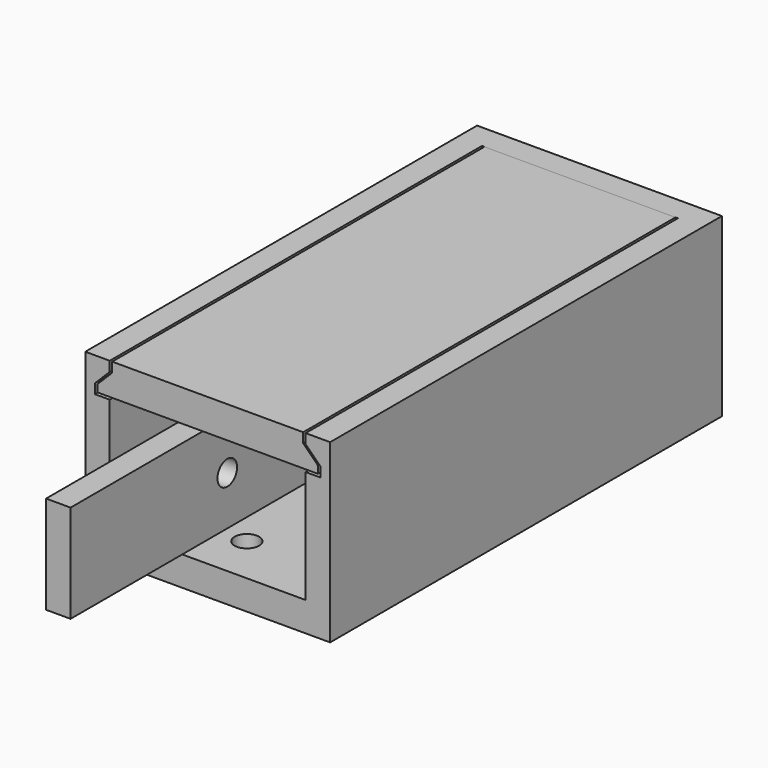
from build123d import *

# Parameters (mm, degrees)
F0_W      = 50
F0_H      = 100
F1_DEPTH  = 6
F3_DEPTH  = 30
F5_DEPTH  = 95
F8_R      = 2.5
F9_DEPTH  = 6
F10_R     = 5
F11_DEPTH = 5
F12_DEPTH = 95
F14_R     = 2.5
F15_DEPTH = 20
F16_R     = 2.5
F17_DEPTH = 5
F16_R_2   = 2.75
F18_DEPTH = 3
F19_DEPTH = 20


# Not quite as in the source:
# - a feature names something its author has since deleted; it is built from what else it names


with BuildPart() as f1:
    # F0 (on Top) → F1 (new body)
    with BuildSketch(Plane.XY):
        Rectangle(F0_W, F0_H)
    extrude(amount=F1_DEPTH)

    # F2 (on face) → F3 (join)
    with BuildSketch(Plane.XY.offset(6)):
        Polygon((-20, 50), (-25, 50), (-25, 45), (-25, -50), (-20, -50), (-20, 45), (20, 45), (20, -50), (25, -50), (25, 45), (25, 50), (20, 50), align=None)
    extrude(amount=F3_DEPTH)

    # F4 (on face) → F5 (cut)
    with BuildSketch(Plane.XZ.offset(50)):
        Polygon((-23, 29), (-20, 29), (-20, 34), (-23, 31), align=None)
        Polygon((20, 34), (20, 29), (23, 29), (23, 31), align=None)
    extrude(amount=-F5_DEPTH, mode=Mode.SUBTRACT)

    # F8 (on face) → F9 (cut, through all)
    with BuildSketch(Plane.XY.offset(6)):
        with Locations((0, -40)):
            Circle(F8_R)
        with Locations((-9, 30)):
            Circle(F8_R)
        with Locations((9, 30)):
            Circle(F8_R)
    extrude(amount=-F9_DEPTH, mode=Mode.SUBTRACT)

    # F10 (on face) → F11 (cut, through all)
    with BuildSketch(Plane(origin=(0, 50, 0), x_dir=(-1, 0, 0), z_dir=(0, 1, 0))):
        with Locations((0, 16)):
            Circle(F10_R)
    extrude(amount=-F11_DEPTH, mode=Mode.SUBTRACT)

    # F8 (on face) → F19 (join)
    with BuildSketch(Plane.XY.offset(6)):
        with Locations((-12, -30)):
            Circle(F8_R)
        with Locations((12, -30)):
            Circle(F8_R)
    extrude(amount=F19_DEPTH)


with BuildPart() as f12:
    # F7 (on offset) → F12 (new body)
    with BuildSketch(Plane.XZ.offset(50)):
        Polygon((-22.5, 31), (-22.5, 29.5), (22.5, 29.5), (22.5, 31), (19.5, 34), (19.5, 36), (-19.5, 36), (-19.5, 34), align=None)
    extrude(amount=-F12_DEPTH)


with BuildPart() as f15:
    # F14 (on offset) → F15 (new body)
    with BuildSketch(Plane.XY.offset(27)):
        with BuildLine():
            Line((-4, -80), (-4, 30))
            ThreePointArc((-4, 30), (-12.5355339059, 33.5355339059), (-9, 25))
            Line((-9, 25), (-9, -80))
            Line((-9, -80), (-4, -80))
        make_face()
        with Locations((-9, 30)):
            Circle(F14_R, mode=Mode.SUBTRACT)
    extrude(amount=-F15_DEPTH)

    # F16 (on face) → F17 (cut, through all)
    with BuildSketch(Plane.YZ.offset(-4)):
        with Locations((-40, 17)):
            Circle(F16_R)
    extrude(amount=-F17_DEPTH, mode=Mode.SUBTRACT)

    # F16 (on face) → F18 (cut)
    with BuildSketch(Plane.YZ.offset(-4)):
        with Locations((5, 17)):
            Circle(F16_R_2)
    extrude(amount=-F18_DEPTH, mode=Mode.SUBTRACT)


solid = Compound([f1.part, f12.part, f15.part])
